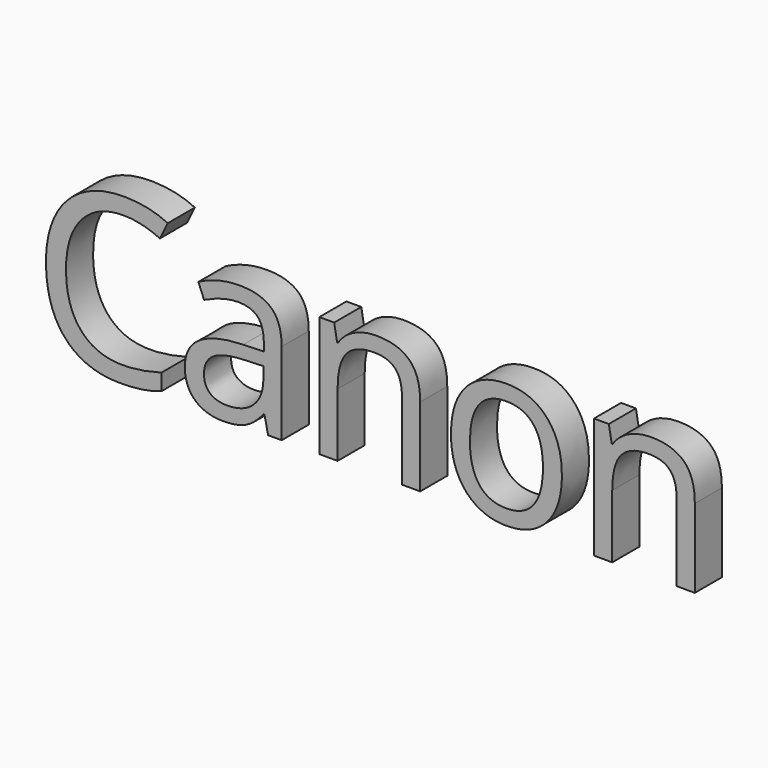
from build123d import *

# Parameters (mm, degrees)
F0_TEXT_SIZE = 8.4582964774
F1_DEPTH     = 1.27


# Not quite as in the source:
# - Text() gives the source's letters only with a copy of the font that has no kerning and outlines rounded to 1/6400 em; it was checked with that copy


with BuildPart() as f1:
    # F0 (on Front) → F1 (new body)
    with BuildSketch(Plane.XZ):
        with Locations((-18.4354105566, 9.3004492391)):
            Text('Canon', F0_TEXT_SIZE, font='Open Sans', text_align=(TextAlign.LEFT, TextAlign.BOTTOM))
    extrude(amount=F1_DEPTH)


solid = f1.part
